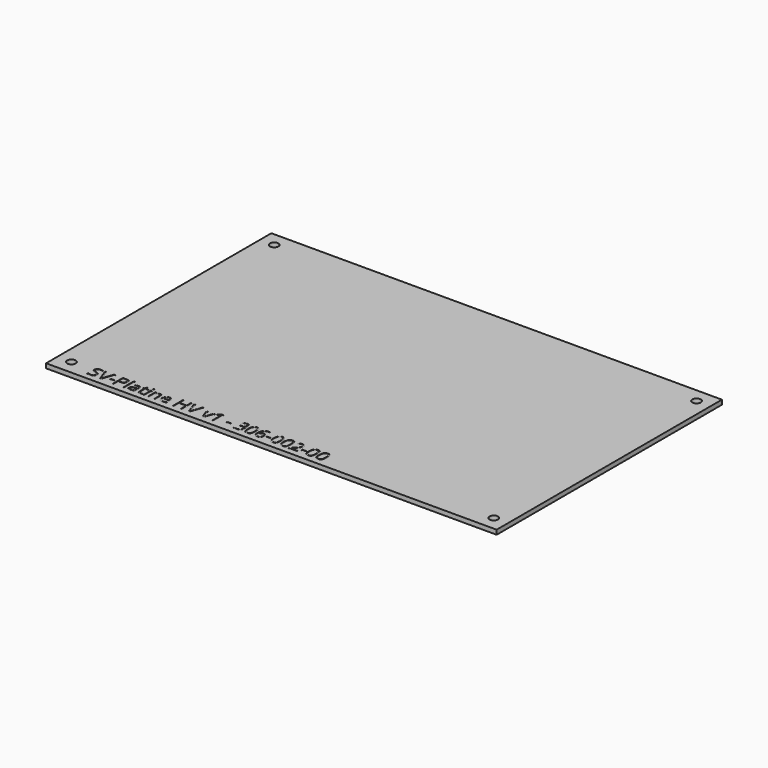
from build123d import *

# Parameters (mm, degrees)
F0_W         = 160
F0_H         = 100
F0_R         = 1.5
F1_DEPTH     = 1.6
F2_TEXT_SIZE = 6.1743944469
F3_DEPTH     = 0.1


# Not quite as in the source:
# - Text() gives the source's letters only with a copy of the font that has no kerning and outlines rounded to 1/6400 em; it was checked with that copy


with BuildPart() as f1:
    # F0 (on Top) → F1 (new body)
    with BuildSketch(Plane.XY):
        Rectangle(F0_W, F0_H)
        with Locations((-75, -45)):
            Circle(F0_R, mode=Mode.SUBTRACT)
        with Locations((75, -45)):
            Circle(F0_R, mode=Mode.SUBTRACT)
        with Locations((-75, 45)):
            Circle(F0_R, mode=Mode.SUBTRACT)
        with Locations((75, 45)):
            Circle(F0_R, mode=Mode.SUBTRACT)
    extrude(amount=-F1_DEPTH)

    # F2 (on face) → F3 (cut)
    with BuildSketch(Plane.XY):
        with Locations((-67.519094795, -47.9870345443)):
            Text('SV-Platine HV v1 - 306-002-00', F2_TEXT_SIZE, font='Open Sans', text_align=(TextAlign.LEFT, TextAlign.BOTTOM))
    extrude(amount=-F3_DEPTH, mode=Mode.SUBTRACT)


solid = f1.part
